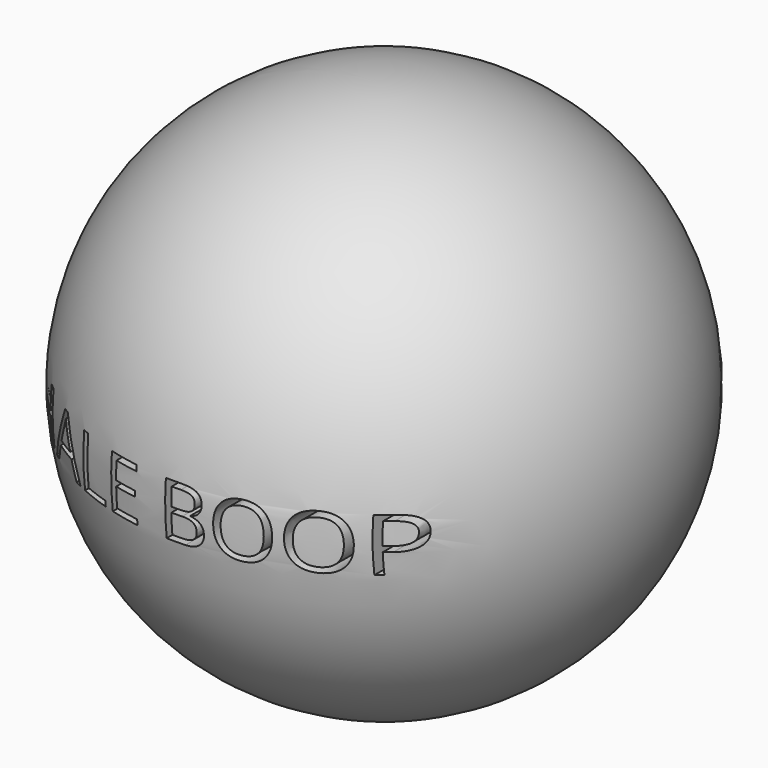
from build123d import *

# Parameters (mm, degrees)
F2_TEXT_SIZE = 22.9792768087
F3_DEPTH     = 254


# Not quite as in the source:
# - Text() gives the source's letters only with a copy of the font that has no kerning and outlines rounded to 1/6400 em; it was checked with that copy


with BuildPart() as f1:
    # F0 (on Front) → F1 (revolve)
    with BuildSketch(Plane.XZ):
        with BuildLine():
            Line((0, -80.7485272673), (0, 80.7485272673))
            ThreePointArc((0, 80.7485272673), (-80.7485272673, 0), (0, -80.7485272673))
        make_face()
    revolve(axis=Axis((0, 0, 0), (0, 0, 1)))

    # F2 (on Front) → F3 (cut, symmetric)
    with BuildSketch(Plane.XZ):
        with Locations((-66.8844782551, -9.7679723104)):
            Text('HALE BOOP', F2_TEXT_SIZE, font='Open Sans', text_align=(TextAlign.LEFT, TextAlign.BOTTOM))
    extrude(amount=F3_DEPTH, both=True, mode=Mode.SUBTRACT)


solid = f1.part
